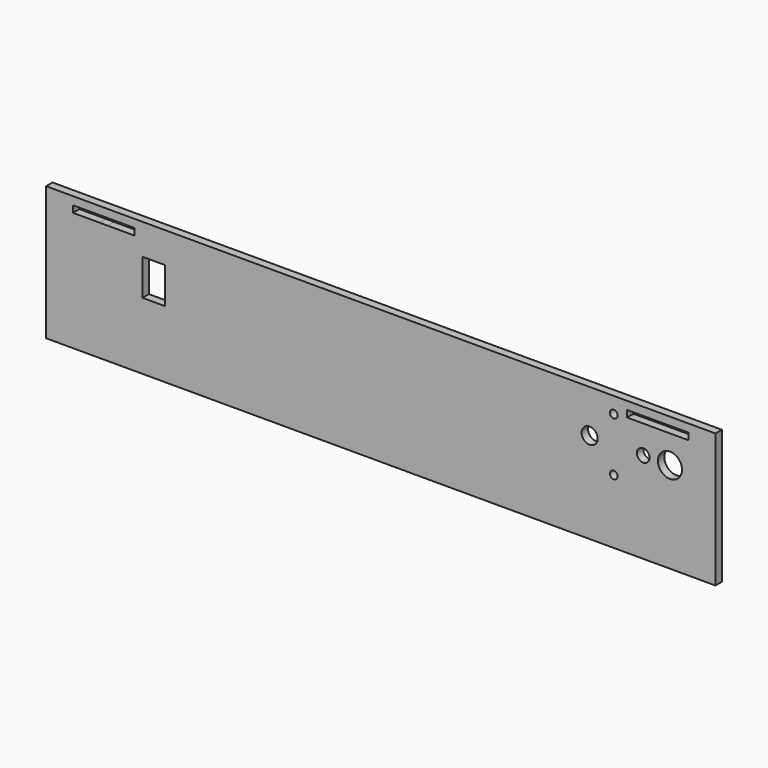
from build123d import *

# Parameters (mm, degrees)
F0_W     = 250
F0_H     = 50
F1_DEPTH = 3
F2_DEPTH = 3
F3_R     = 4.5
F3_R_2   = 1.45
F3_R_3   = 2.375
F3_R_4   = 3
F3_W     = 8.5
F3_H     = 13.5
F4_DEPTH = 25


# Not quite as in the source:
# - ends of sketch curves that miss each other by under 0.0002 mm in the source are joined


with BuildPart() as f1:
    # F0 (on Front) → F1 (new body)
    with BuildSketch(Plane.XZ):
        with Locations((-42.7222467884, 16.2994446903)):
            Rectangle(F0_W, F0_H)
        Polygon((-147.7222467884, 35.7994452119), (-157.7222467884, 35.7994452119), (-157.7222467884, 38.2994446903), (-134.7222467884, 38.2994446903), (-134.7222467884, 35.7994446903), (-144.7222467884, 35.7994446903), align=None, mode=Mode.SUBTRACT)
        Polygon((49.2777532116, 38.2994446903), (62.2777532116, 38.2994446903), (72.2777532116, 38.2994446903), (72.2777532116, 35.7994446903), (49.2777532116, 35.7994446903), align=None, mode=Mode.SUBTRACT)
    extrude(amount=F1_DEPTH)

    # F0 (on Front) → F2 (join)
    with BuildSketch(Plane.XZ):
        with Locations((-42.7222467884, 16.2994446903)):
            Rectangle(F0_W, F0_H)
        Polygon((-147.7222467884, 35.7994452119), (-157.7222467884, 35.7994452119), (-157.7222467884, 38.2994446903), (-134.7222467884, 38.2994446903), (-134.7222467884, 35.7994446903), (-144.7222467884, 35.7994446903), align=None, mode=Mode.SUBTRACT)
        Polygon((49.2777532116, 38.2994446903), (62.2777532116, 38.2994446903), (72.2777532116, 38.2994446903), (72.2777532116, 35.7994446903), (49.2777532116, 35.7994446903), align=None, mode=Mode.SUBTRACT)
    extrude(amount=F2_DEPTH)

    # F3 (on face) → F4 (cut)
    with BuildSketch(Plane(origin=(0, 0, 0), x_dir=(-1, 0, 0), z_dir=(0, 1, 0))):
        with Locations((-65.2777532116, 25.2994446903)):
            Circle(F3_R)
        with Locations((-44.2777532116, 15.2994446903)):
            Circle(F3_R_2)
        with Locations((-44.2777532116, 35.2994446903)):
            Circle(F3_R_2)
        with Locations((-55.2777532116, 25.2994446903)):
            Circle(F3_R_3)
        with Locations((-35.2777532116, 25.2994446903)):
            Circle(F3_R_4)
        with Locations((127.4722467884, 23.0494446903)):
            Rectangle(F3_W, F3_H)
    extrude(amount=-F4_DEPTH, mode=Mode.SUBTRACT)


solid = f1.part
